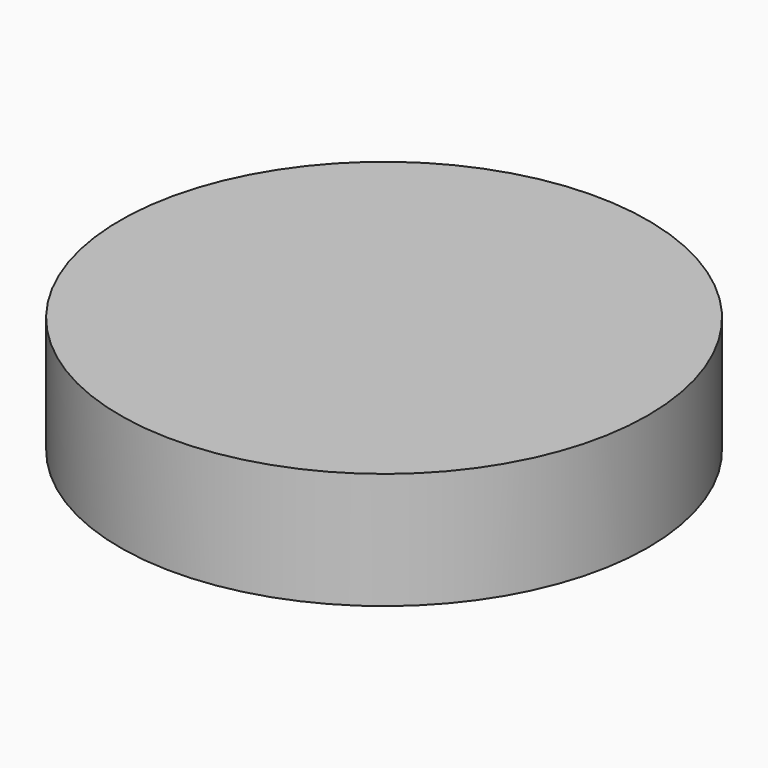
from build123d import *

# Parameters (mm, degrees)
F0_R     = 57.5961395205
F1_DEPTH = 25.4
F2_R     = 41.9082998656
F3_DEPTH = 178
F4_R     = 11.649028694
F5_DEPTH = 12.7


# Not quite as in the source:
# - an extrude ends at something that could not be found from the text; its depth is read off the source's solid


with BuildPart() as f1:
    # F0 (on Top) → F1 (new body)
    with BuildSketch(Plane.XY):
        Circle(F0_R)
    extrude(amount=F1_DEPTH)

    # F2 (on Top) → F3 (cut, through all)
    with BuildSketch(Plane.XY):
        Circle(F2_R)
    extrude(amount=-F3_DEPTH, mode=Mode.SUBTRACT)

    # F4 (on Front) → F5 (cut)
    with BuildSketch(Plane.XZ):
        with Locations((-8.324730893, 12.7451797782)):
            Circle(F4_R)
    extrude(amount=-F5_DEPTH, mode=Mode.SUBTRACT)


solid = f1.part
